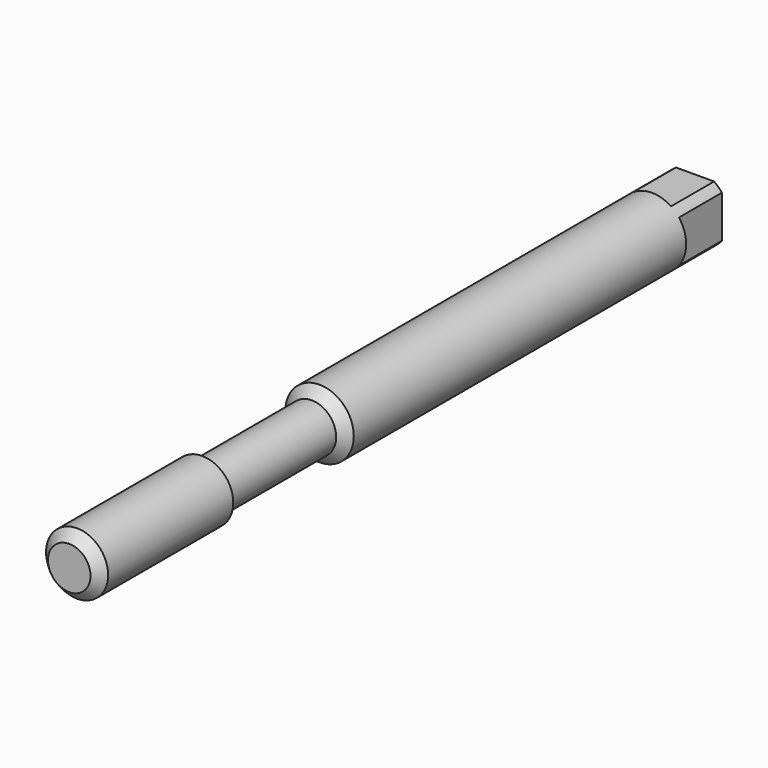
from build123d import *

# Parameters (mm, degrees)
F0_R        = 3.5
F1_DEPTH    = 80
F2_R        = 6.3298520118
F2_R_2      = 2.5
F3_DEPTH    = 30
F4_S5_R     = 2.5
F4_T6_DEPTH = 7
F5_R        = 3.175
F6_DEPTH    = 17
F7_SIZE     = 1
F8_W        = 9.7203729674
F8_H        = 8.019306697
F8_W_2      = 5.5
F8_H_2      = 5.8197690165
F9_DEPTH    = 5.5


# Not quite as in the source:
# - a fillet or chamfer that OpenCascade refuses, or shapes differently, is made with other operations: its cross-section is extruded or revolved along the edge and cut away or added


with BuildPart() as f1:
    # F0 (on Front) → F1 (new body)
    with BuildSketch(Plane.XZ):
        Circle(F0_R)
    extrude(amount=F1_DEPTH)

    # F2 (on face) → F3 (cut)
    with BuildSketch(Plane.XZ.offset(80)):
        Circle(F2_R)
        Circle(F2_R_2, mode=Mode.SUBTRACT)
    extrude(amount=-F3_DEPTH, mode=Mode.SUBTRACT)

    # F4: chamfer of 2 on 1 edges, made by hand


with BuildPart() as f4_tool2:
    # F4_s3 → F4_t4 (revolve)
    with BuildSketch(Plane.XY):
        Polygon((3.5, -48), (1.5, -50), (3.5, -50), align=None)
    revolve(axis=Axis((0, -50, 0), (0, 1, 0)))

    # F4_s5 → F4_t6 (cut, symmetric)
    with BuildSketch(Plane.XZ.offset(49)):
        Circle(F4_S5_R)
    extrude(amount=F4_T6_DEPTH, both=True, mode=Mode.SUBTRACT)


with BuildPart() as f1_1:
    add(f1.part)

    # F4_t1: cut F4_tool2
    add(f4_tool2.part, mode=Mode.SUBTRACT)

    # F5 (on face) → F6 (join)
    with BuildSketch(Plane.XZ.offset(80)):
        Circle(F5_R)
    extrude(amount=-F6_DEPTH)

    # F7
    f7_edges = [f1_1.edges().sort_by_distance(p)[0] for p in [
        (-3.175, -80, 0),
    ]]
    chamfer(f7_edges, length=F7_SIZE)

    # F8 (on face) → F9 (cut)
    with BuildSketch(Plane(origin=(0, 0, 0), x_dir=(-1, 0, 0), z_dir=(0, 1, 0))):
        Rectangle(F8_W, F8_H)
        Rectangle(F8_W_2, F8_H_2, mode=Mode.SUBTRACT)
    extrude(amount=-F9_DEPTH, mode=Mode.SUBTRACT)


solid = f1_1.part
